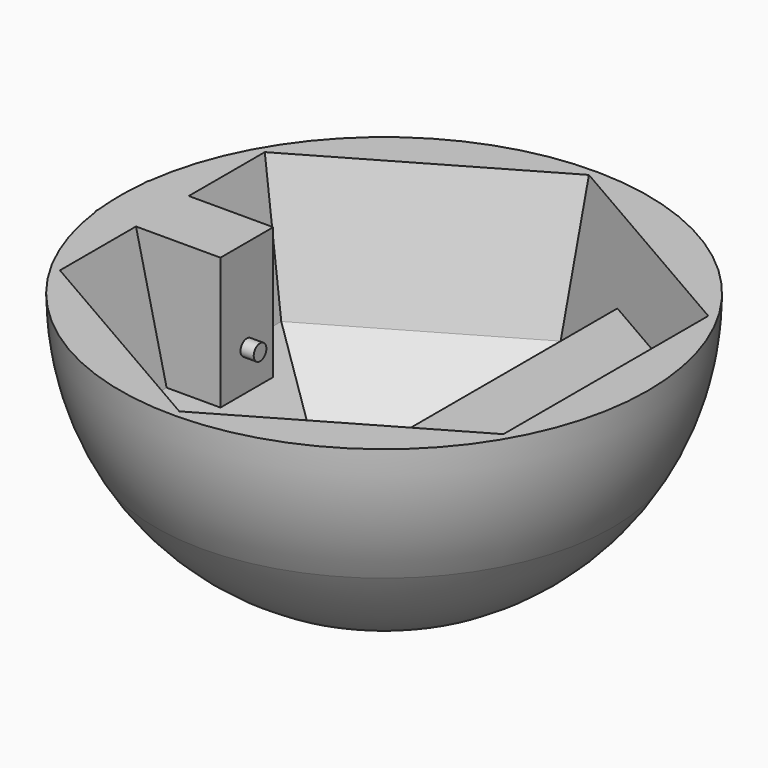
from build123d import *

# Parameters (mm, degrees)
F11_W      = 36.5
F11_H      = 3
F15_DEPTH  = 12.5
F16_R      = 3
F17_DEPTH  = 5
F18_W      = 36.5
F18_H      = 3
F19_FACE_W = 36.5
F19_FACE_H = 3


with BuildPart() as f1:
    # F0 (on Front) → F1 (revolve)
    with BuildSketch(Plane.XZ):
        with BuildLine():
            Line((0, -50), (-86.6025403784, -50))
            ThreePointArc((-86.6025403784, -50), (-50, -86.6025403784), (0, -100))
            Line((0, -100), (0, -50))
        make_face()
    revolve(axis=Axis((0, 0, -75), (0, 0, -1)))

    # F3 (on face) → F6 section 0
    with BuildSketch(Plane.XY.offset(-50)):
        Polygon((0, -83.6025403784), (72.4019237886, -41.8012701892), (72.4019237886, 41.8012701892), (0, 83.6025403784), (-72.4019237886, 41.8012701892), (-72.4019237886, -41.8012701892), align=None)
    # F5 (on offset) → F6 section 1
    with BuildSketch(Plane.XY.offset(-85)):
        Polygon((45.0333209968, 26), (0, 52), (-45.0333209968, 26), (-45.0333209968, -26), (0, -52), (45.0333209968, -26), align=None)
    loft(mode=Mode.SUBTRACT)

    # F11 (on Front) → F12 (join, up to the last surface of F1)
    with BuildSketch(Plane.XZ):
        with Locations((-26.7833209968, -76.5)):
            Rectangle(F11_W, F11_H)
    extrude(until=Until.LAST)

    # F11 (on Front) → F13 (join, up to the last surface of F1)
    with BuildSketch(Plane.XZ):
        with Locations((-26.7833209968, -76.5)):
            Rectangle(F11_W, F11_H)
    extrude(until=Until.LAST, dir=(0, 1, 0))


with BuildPart() as f8:
    # F7 (on Front) → F8 (revolve)
    with BuildSketch(Plane.XZ):
        with BuildLine():
            ThreePointArc((-100, 0), (-96.5925826289, -25.8819045103), (-86.6025403784, -50))
            Line((-86.6025403784, -50), (0, -50))
            Line((0, -50), (0, 0))
            Line((0, 0), (-100, 0))
        make_face()
    revolve(axis=Axis((0, 0, -25), (0, 0, -1)))

    # F9 (on face) → F10 section 0
    with BuildSketch(Plane.XY):
        Polygon((0, -97), (84.0044641671, -48.5), (84.0044641671, 48.5), (0, 97), (-84.0044641671, 48.5), (-84.0044641671, -48.5), align=None)
    # F3 (on face) → F10 section 1
    with BuildSketch(Plane.XY.offset(-50)):
        Polygon((0, -83.6025403784), (72.4019237886, -41.8012701892), (72.4019237886, 41.8012701892), (0, 83.6025403784), (-72.4019237886, 41.8012701892), (-72.4019237886, -41.8012701892), align=None)
    loft(mode=Mode.SUBTRACT)

    # F14 (on Front) → F15 (join, symmetric)
    with BuildSketch(Plane.XZ):
        Polygon((-52, 0), (-99.4761735201, 0), (-72.4019237886, -50), (-52, -50), align=None)
    extrude(amount=F15_DEPTH, both=True)

    # F16 (on face) → F17 (join)
    with BuildSketch(Plane.YZ.offset(-52)):
        with Locations((0, -35)):
            Circle(F16_R)
    extrude(amount=F17_DEPTH)

    # F18 (on Front) → F19 (join, up to the last surface of F8)
    with BuildSketch(Plane.XZ):
        with Locations((48.25, -26.5)):
            Rectangle(F18_W, F18_H)
    extrude(until=Until.LAST)

    # F19_face (on face) → F20 (join, up to the last surface of F8)
    with BuildSketch(Plane(origin=(48.25, 0, -26.5), x_dir=(1, 0, 0), z_dir=(0, 1, 0))):
        Rectangle(F19_FACE_W, F19_FACE_H)
    extrude(until=Until.LAST)


solid = Compound([f1.part, f8.part])
